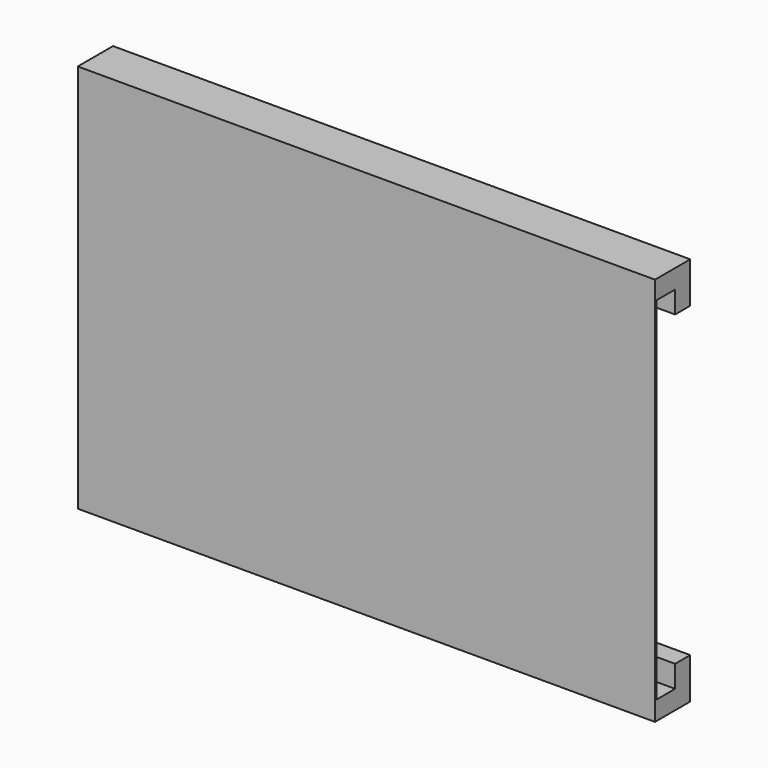
from build123d import *

# Parameters (mm, degrees)
F0_W          = 410
F0_H          = 335
F0_W_2        = 385
F0_H_2        = 310
F1_DEPTH      = 22
F2_DEPTH      = 20
F4_DEPTH      = 480
F4_DEPTH_BACK = 70
F5_W          = 366
F5_H          = 239
F6_DEPTH      = 30
F7_R          = 29.99999
F9_W          = 550
F9_H          = 371
F10_DEPTH     = 2


# Not quite as in the source:
# - a fillet or chamfer is up to 0.001 mm smaller than in the source, because OpenCascade refuses the exact size


with BuildPart() as f1:
    # F0 (on Front) → F1 (new body)
    with BuildSketch(Plane.XZ):
        Rectangle(F0_W, F0_H)
        Rectangle(F0_W_2, F0_H_2, mode=Mode.SUBTRACT)
    extrude(amount=F1_DEPTH)

    # F0 (on Front) → F2 (join)
    with BuildSketch(Plane.XZ):
        Rectangle(F0_W_2, F0_H_2)
    extrude(amount=F2_DEPTH)

    # F5 (on face) → F6 (join)
    with BuildSketch(Plane(origin=(0, 0, 0), x_dir=(-1, 0, 0), z_dir=(0, 1, 0))):
        with Locations((0, 12)):
            Rectangle(F5_W, F5_H)
    extrude(amount=F6_DEPTH)

    # F7 (radius 30 in the source; OpenCascade refuses exactly that, so slightly less here)
    f7_edges = [f1.edges().sort_by_distance(p)[0] for p in [
        (-183, 30, 12),
        (0, 30, 131.5),
        (183, 30, 12),
        (0, 30, -107.5),
    ]]
    fillet(f7_edges, radius=F7_R)


with BuildPart() as f4:
    # F3 (on face) → F4 (new body, two sides)
    with BuildSketch(Plane.YZ.offset(205)) as f4_sk:
        Polygon((0, -167.5), (-22, -167.5), (-22, -185.5), (18, -185.5), (18, -146.5062479338), (0, -146.5062479338), align=None)
    extrude(amount=-F4_DEPTH)
    extrude(f4_sk.sketch, amount=F4_DEPTH_BACK)


with BuildPart() as f4b:
    # F3 (on face) → F4, piece 2 (new body, two sides)
    with BuildSketch(Plane.YZ.offset(205)) as f4_2_sk:
        Polygon((0, 146.5062479338), (18, 146.5062479338), (18, 185.5), (-22, 185.5), (-22, 167.5), (0, 167.5), align=None)
    extrude(amount=-F4_DEPTH)
    extrude(f4_2_sk.sketch, amount=F4_DEPTH_BACK)


with BuildPart() as f4_1:
    add(f4.part)

    # F8: union F4b, F1
    add(f4b.part)
    add(f1.part)

    # F9 (on face) → F10 (join)
    with BuildSketch(Plane.XZ.offset(22)):
        Rectangle(F9_W, F9_H)
    extrude(amount=F10_DEPTH)


solid = f4_1.part
